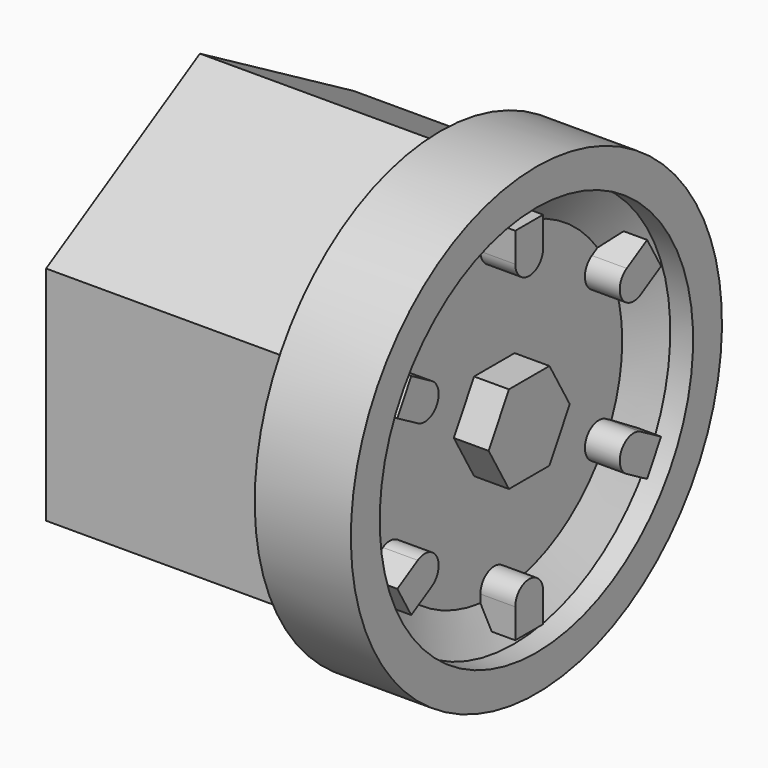
from build123d import *

# Parameters (mm, degrees)
F3_DEPTH        = 2.9
F5_DEPTH        = 20
F7_DEPTH        = 2.9
F7_COPIES_COUNT = 6


# Not quite as in the source:
# - a pattern or mirror of a feature is missing from the dataset's text; its kind, count and spacing are read off the source's solid


with BuildPart() as f1:
    # F0 (on Front) → F1 (revolve)
    with BuildSketch(Plane.XZ):
        Polygon((1.6, 16.3), (3.5, 16.3), (3.5, 19.3), (-4.5, 19.3), (-4.5, 0), (0, 0), (0, 13.3), align=None)
    revolve(axis=Axis((15.3209697455, 0, 0), (1, 0, 0)))

    # F2 (on face) → F3 (join)
    with BuildSketch(Plane.YZ):
        Polygon((-2.1073284825, 3.65), (-4.2146569651, 0), (-2.1073284825, -3.65), (2.1073284825, -3.65), (4.2146569651, 0), (2.1073284825, 3.65), align=None)
    extrude(amount=F3_DEPTH)

    # F4 (on face) → F5 (join)
    with BuildSketch(Plane(origin=(-4.5, 0, 0), x_dir=(0, -1, 0), z_dir=(-1, 0, 0))):
        Polygon((0, 18.4752086141), (-16, 9.237604307), (-16, -9.237604307), (0, -18.4752086141), (16, -9.237604307), (16, 9.237604307), align=None)
    extrude(amount=F5_DEPTH)

    # F6 (on face) → F7 (join)
    with BuildSketch(Plane.YZ):
        with BuildLine():
            Line((1.45, 15), (-1.45, 15))
            Line((-1.45, 15), (-1.45, 12.55))
            ThreePointArc((-1.45, 12.55), (0, 11.1), (1.45, 12.55))
            Line((1.45, 12.55), (1.45, 15))
        make_face()
    f7 = extrude(amount=F7_DEPTH)

    # F7_copies: F7 ×6 about axis
    f7_copies_axis = Axis((0, 0, 0), (1, 0, 0))
    for i in range(1, F7_COPIES_COUNT):
        add(f7.rotate(f7_copies_axis, i * 360 / F7_COPIES_COUNT))


solid = f1.part
